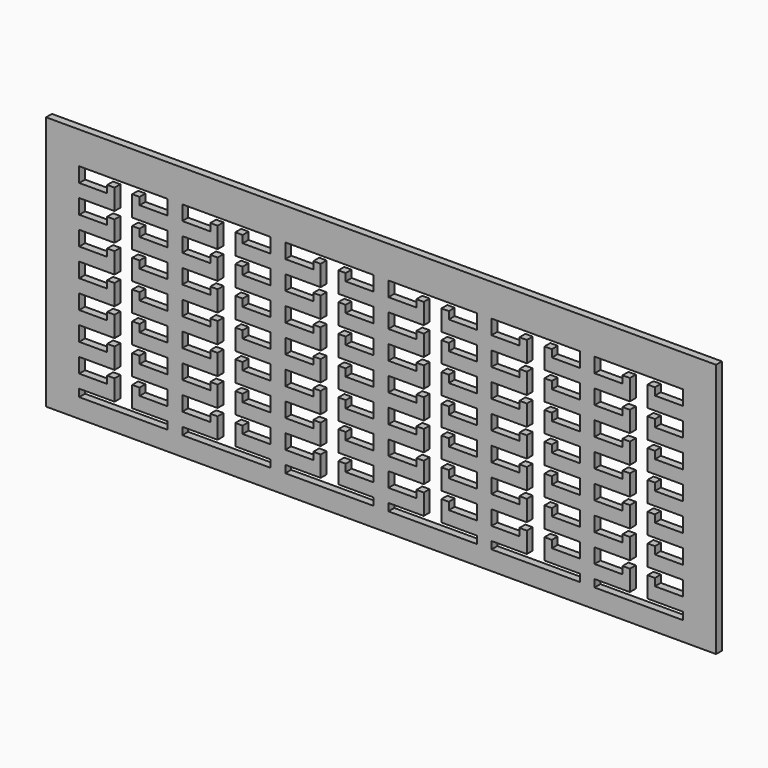
from build123d import *

# Parameters (mm, degrees)
F0_W     = 577.85
F0_H     = 219.71
F1_DEPTH = 6.35


# Not quite as in the source:
# - ends of sketch curves that miss each other by under 0.0002 mm in the source are joined


with BuildPart() as f1:
    # F0 (on Front) → F1 (new body)
    with BuildSketch(Plane.XZ):
        with Locations((-282.1097705345, 13.2987275338)):
            Rectangle(F0_W, F0_H)
        Polygon((-542.4597705345, -62.2027724662), (-542.4597705345, -49.5027724662), (-511.9797705345, -49.5027724662), (-511.9797705345, -31.7227724662), (-518.3297705345, -31.7227724662), (-518.3297705345, -38.0727724662), (-542.4597705345, -38.0727724662), (-542.4597705345, -25.3727724662), (-511.9797705345, -25.3727724662), (-511.9797705345, -7.5927724662), (-518.3297705345, -7.5927724662), (-518.3297705345, -13.9427724662), (-542.4597705345, -13.9427724662), (-542.4597705345, -1.2427724662), (-511.9797705345, -1.2427724662), (-511.9797705345, 16.5372275338), (-518.3297705345, 16.5372275338), (-518.3297705345, 10.1872275338), (-542.4597705345, 10.1872275338), (-542.4597705345, 22.8872275338), (-511.9797705345, 22.8872275338), (-511.9797705345, 40.6672275338), (-518.3297705345, 40.6672275338), (-518.3297705345, 34.3172275338), (-542.4597705345, 34.3172275338), (-542.4597705345, 47.0172275338), (-511.9797705345, 47.0172275338), (-511.9797705345, 64.7972275338), (-518.3297705345, 64.7972275338), (-518.3297705345, 58.4472275338), (-542.4597705345, 58.4472275338), (-542.4597705345, 71.1472275338), (-511.9797705345, 71.1472275338), (-511.9797705345, 88.9272173567), (-518.3297705345, 88.9272173567), (-518.3297705345, 82.5772173567), (-542.4597705345, 82.5772173567), (-542.4597705345, 95.2772173567), (-466.2597705346, 95.2772173567), (-466.2597705346, 82.5772173567), (-490.3897705345, 82.5772173567), (-490.3897705345, 88.9272173567), (-496.7397705346, 88.9272173567), (-496.7397705346, 71.1472173567), (-466.2597705346, 71.1472173568), (-466.2597705346, 58.4472173568), (-490.3897705346, 58.4472173568), (-490.3897705346, 64.7972173568), (-496.7397705346, 64.7972173568), (-496.7397705346, 47.0172173567), (-466.2597705346, 47.0172173567), (-466.2597705345, 34.3172275338), (-490.3897705345, 34.3172275338), (-490.3897705345, 40.6672275338), (-496.7397705345, 40.6672275338), (-496.7397705345, 22.8872275338), (-466.2597705345, 22.8872275338), (-466.2597705345, 10.1872275338), (-490.3897705345, 10.1872275338), (-490.3897705345, 16.5372275338), (-496.7397705345, 16.5372275338), (-496.7397705345, -1.2427724662), (-466.2597705345, -1.2427724662), (-466.2597705345, -13.9427724662), (-490.3897705345, -13.9427724662), (-490.3897705345, -7.5927724662), (-496.7397705345, -7.5927724662), (-496.7397705345, -25.3727724662), (-466.2597705345, -25.3727724662), (-466.2597705345, -38.0727724662), (-490.3897705345, -38.0727724662), (-490.3897705345, -31.7227724662), (-496.7397705345, -31.7227724662), (-496.7397705345, -49.5027724662), (-466.2597705345, -49.5027724662), (-466.2597705345, -62.2027724662), (-490.3897705345, -62.2027724662), (-490.3897705345, -55.8527724662), (-496.7397705345, -55.8527724662), (-496.7397705345, -73.6327724662), (-466.2597705345, -73.6327724662), (-466.2597705345, -80.0462724662), (-542.4597705345, -80.0462724662), (-542.4597705345, -73.6327724662), (-511.9797705345, -73.6327724662), (-511.9797705345, -55.8527724662), (-518.3297705345, -55.8527724662), (-518.3297705345, -62.2027724662), align=None, mode=Mode.SUBTRACT)
        Polygon((-453.5597705345, -62.2027724662), (-453.5597705345, -49.5027724662), (-423.0797705345, -49.5027724662), (-423.0797705345, -31.7227724662), (-429.4297705345, -31.7227724662), (-429.4297705345, -38.0727724662), (-453.5597705345, -38.0727724662), (-453.5597705345, -25.3727724662), (-423.0797705345, -25.3727724662), (-423.0797705345, -7.5927724662), (-429.4297705345, -7.5927724662), (-429.4297705345, -13.9427724662), (-453.5597705345, -13.9427724662), (-453.5597705345, -1.2427724662), (-423.0797705345, -1.2427724662), (-423.0797705345, 16.5372275338), (-429.4297705345, 16.5372275338), (-429.4297705345, 10.1872275338), (-453.5597705345, 10.1872275338), (-453.5597705345, 22.8872275338), (-423.0797705345, 22.8872275338), (-423.0797705345, 40.6672275338), (-429.4297705345, 40.6672275338), (-429.4297705345, 34.3172275338), (-453.5597705345, 34.3172275338), (-453.5597705345, 47.0172275338), (-423.0797705345, 47.0172275338), (-423.0797705345, 64.7972275338), (-429.4297705345, 64.7972275338), (-429.4297705345, 58.4472275338), (-453.5597705345, 58.4472275338), (-453.5597705345, 71.1472275338), (-423.0797705345, 71.1472275338), (-423.0797705345, 88.9272275338), (-429.4297705345, 88.9272275338), (-429.4297705345, 82.5772275338), (-453.5597705345, 82.5772275338), (-453.5597705345, 95.2772275338), (-377.3597705345, 95.2772275338), (-377.3597705345, 82.5772275338), (-401.4897705345, 82.5772275338), (-401.4897705345, 88.9272275338), (-407.8397705345, 88.9272275338), (-407.8397705345, 71.1472275338), (-377.3597705345, 71.1472275338), (-377.3597705345, 58.4472275338), (-401.4897705345, 58.4472275338), (-401.4897705345, 64.7972275338), (-407.8397705345, 64.7972275338), (-407.8397705345, 47.0172275338), (-377.3597705345, 47.0172275338), (-377.3597705345, 34.3172275338), (-401.4897705345, 34.3172275338), (-401.4897705345, 40.6672275338), (-407.8397705345, 40.6672275338), (-407.8397705345, 22.8872275338), (-377.3597705345, 22.8872275338), (-377.3597705345, 10.1872275338), (-401.4897705345, 10.1872275338), (-401.4897705345, 16.5372275338), (-407.8397705345, 16.5372275338), (-407.8397705345, -1.2427724662), (-377.3597705345, -1.2427724662), (-377.3597705345, -13.9427724662), (-401.4897705345, -13.9427724662), (-401.4897705345, -7.5927724662), (-407.8397705345, -7.5927724662), (-407.8397705345, -25.3727724662), (-377.3597705345, -25.3727724662), (-377.3597705345, -38.0727724662), (-401.4897705345, -38.0727724662), (-401.4897705345, -31.7227724662), (-407.8397705345, -31.7227724662), (-407.8397705345, -49.5027724662), (-377.3597705345, -49.5027724662), (-377.3597705345, -62.2027724662), (-401.4897705345, -62.2027724662), (-401.4897705345, -55.8527724662), (-407.8397705345, -55.8527724662), (-407.8397705345, -73.6327724662), (-377.3597705345, -73.6327724662), (-377.3597705345, -80.0462724662), (-453.5597705345, -80.0462724662), (-453.5597705345, -73.6327724662), (-423.0797705345, -73.6327724662), (-423.0797705345, -55.8527724662), (-429.4297705345, -55.8527724662), (-429.4297705345, -62.2027724662), align=None, mode=Mode.SUBTRACT)
        Polygon((-364.6597705345, -62.2027724662), (-364.6597705345, -49.5027724662), (-334.1797705345, -49.5027724662), (-334.1797705345, -31.7227724662), (-340.5297705345, -31.7227724662), (-340.5297705345, -38.0727724662), (-364.6597705345, -38.0727724662), (-364.6597705345, -25.3727724662), (-334.1797705345, -25.3727724662), (-334.1797705345, -7.5927724662), (-340.5297705345, -7.5927724662), (-340.5297705345, -13.9427724662), (-364.6597705345, -13.9427724662), (-364.6597705345, -1.2427724662), (-334.1797705345, -1.2427724662), (-334.1797705345, 16.5372275338), (-340.5297705345, 16.5372275338), (-340.5297705345, 10.1872275338), (-364.6597705345, 10.1872275338), (-364.6597705345, 22.8872275338), (-334.1797705345, 22.8872275338), (-334.1797705345, 40.6672275338), (-340.5297705345, 40.6672275338), (-340.5297705345, 34.3172275338), (-364.6597705345, 34.3172275338), (-364.6597705345, 47.0172275338), (-334.1797705345, 47.0172275338), (-334.1797705345, 64.7972275338), (-340.5297705345, 64.7972275338), (-340.5297705345, 58.4472275338), (-364.6597705345, 58.4472275338), (-364.6597705345, 71.1472275338), (-334.1797705345, 71.1472275338), (-334.1797705345, 88.9272275338), (-340.5297705345, 88.9272275338), (-340.5297705345, 82.5772275338), (-364.6597705345, 82.5772275338), (-364.6597705345, 95.2772275338), (-288.4597705345, 95.2772275338), (-288.4597705345, 82.5772275338), (-312.5897705345, 82.5772275338), (-312.5897705345, 88.9272275338), (-318.9397705345, 88.9272275338), (-318.9397705345, 71.1472275338), (-288.4597705346, 71.1472275338), (-288.4597705346, 58.4472275338), (-312.5897705346, 58.4472275338), (-312.5897705346, 64.7972275338), (-318.9397705345, 64.7972275338), (-318.9397705346, 47.0172275338), (-288.4597705346, 47.0172275338), (-288.4597705345, 34.3172275338), (-312.5897705345, 34.3172275338), (-312.5897705345, 40.6672275338), (-318.9397705345, 40.6672275338), (-318.9397705345, 22.8872275338), (-288.4597705345, 22.8872275338), (-288.4597705345, 10.1872275338), (-312.5897705345, 10.1872275338), (-312.5897705345, 16.5372275338), (-318.9397705345, 16.5372275338), (-318.9397705345, -1.2427724662), (-288.4597705345, -1.2427724662), (-288.4597705345, -13.9427724662), (-312.5897705345, -13.9427724662), (-312.5897705345, -7.5927724662), (-318.9397705345, -7.5927724662), (-318.9397705345, -25.3727724662), (-288.4597705345, -25.3727724662), (-288.4597705345, -38.0727724662), (-312.5897705345, -38.0727724662), (-312.5897705345, -31.7227724662), (-318.9397705345, -31.7227724662), (-318.9397705345, -49.5027724662), (-288.4597705345, -49.5027724662), (-288.4597705345, -62.2027724662), (-312.5897705345, -62.2027724662), (-312.5897705345, -55.8527724662), (-318.9397705345, -55.8527724662), (-318.9397705345, -73.6327724662), (-288.4597705345, -73.6327724662), (-288.4597705345, -80.0462724662), (-364.6597705345, -80.0462724662), (-364.6597705345, -73.6327724662), (-334.1797705345, -73.6327724662), (-334.1797705345, -55.8527724662), (-340.5297705345, -55.8527724662), (-340.5297705345, -62.2027724662), align=None, mode=Mode.SUBTRACT)
        Polygon((-275.7597705345, -62.2027724662), (-275.7597705345, -49.5027724662), (-245.2797705345, -49.5027724662), (-245.2797705345, -31.7227724662), (-251.6297705345, -31.7227724662), (-251.6297705345, -38.0727724662), (-275.7597705345, -38.0727724662), (-275.7597705345, -25.3727724662), (-245.2797705345, -25.3727724662), (-245.2797705345, -7.5927724662), (-251.6297705345, -7.5927724662), (-251.6297705345, -13.9427724662), (-275.7597705345, -13.9427724662), (-275.7597705345, -1.2427724662), (-245.2797705345, -1.2427724662), (-245.2797705345, 16.5372275338), (-251.6297705345, 16.5372275338), (-251.6297705345, 10.1872275338), (-275.7597705345, 10.1872275338), (-275.7597705345, 22.8872275338), (-245.2797705345, 22.8872275338), (-245.2797705345, 40.6672275338), (-251.6297705345, 40.6672275338), (-251.6297705345, 34.3172275338), (-275.7597705345, 34.3172275338), (-275.7597705345, 47.0172275338), (-245.2797705345, 47.0172275338), (-245.2797705345, 64.7972275338), (-251.6297705345, 64.7972275338), (-251.6297705345, 58.4472275338), (-275.7597705345, 58.4472275338), (-275.7597705345, 71.1472275338), (-245.2797705345, 71.1472275338), (-245.2797705345, 88.9272275338), (-251.6297705345, 88.9272275338), (-251.6297705345, 82.5772275338), (-275.7597705345, 82.5772275338), (-275.7597705345, 95.2772275338), (-199.5597705345, 95.2772275338), (-199.5597705345, 82.5772275338), (-223.6897705345, 82.5772275338), (-223.6897705345, 88.9272275338), (-230.0397705345, 88.9272275338), (-230.0397705345, 71.1472275338), (-199.5597705345, 71.1472275338), (-199.5597705345, 58.4472275338), (-223.6897705345, 58.4472275338), (-223.6897705345, 64.7972275338), (-230.0397705345, 64.7972275338), (-230.0397705345, 47.0172275338), (-199.5597705345, 47.0172275338), (-199.5597705345, 34.3172275338), (-223.6897705345, 34.3172275338), (-223.6897705345, 40.6672275338), (-230.0397705345, 40.6672275338), (-230.0397705345, 22.8872275338), (-199.5597705345, 22.8872275338), (-199.5597705345, 10.1872275338), (-223.6897705345, 10.1872275338), (-223.6897705345, 16.5372275338), (-230.0397705345, 16.5372275338), (-230.0397705345, -1.2427724662), (-199.5597705345, -1.2427724662), (-199.5597705345, -13.9427724662), (-223.6897705345, -13.9427724662), (-223.6897705345, -7.5927724662), (-230.0397705345, -7.5927724662), (-230.0397705345, -25.3727724662), (-199.5597705345, -25.3727724662), (-199.5597705345, -38.0727724662), (-223.6897705345, -38.0727724662), (-223.6897705345, -31.7227724662), (-230.0397705345, -31.7227724662), (-230.0397705345, -49.5027724662), (-199.5597705345, -49.5027724662), (-199.5597705345, -62.2027724662), (-223.6897705345, -62.2027724662), (-223.6897705345, -55.8527724662), (-230.0397705345, -55.8527724662), (-230.0397705345, -73.6327724662), (-199.5597705345, -73.6327724662), (-199.5597705345, -80.0462724662), (-275.7597705345, -80.0462724662), (-275.7597705345, -73.6327724662), (-245.2797705345, -73.6327724662), (-245.2797705345, -55.8527724662), (-251.6297705345, -55.8527724662), (-251.6297705345, -62.2027724662), align=None, mode=Mode.SUBTRACT)
        Polygon((-186.8597705345, -62.2027724662), (-186.8597705345, -49.5027724662), (-156.3797705345, -49.5027724662), (-156.3797705345, -31.7227724662), (-162.7297705345, -31.7227724662), (-162.7297705345, -38.0727724662), (-186.8597705345, -38.0727724662), (-186.8597705345, -25.3727724662), (-156.3797705345, -25.3727724662), (-156.3797705345, -7.5927724662), (-162.7297705345, -7.5927724662), (-162.7297705345, -13.9427724662), (-186.8597705345, -13.9427724662), (-186.8597705345, -1.2427724662), (-156.3797705345, -1.2427724662), (-156.3797705345, 16.5372275338), (-162.7297705345, 16.5372275338), (-162.7297705345, 10.1872275338), (-186.8597705345, 10.1872275338), (-186.8597705345, 22.8872275338), (-156.3797705345, 22.8872275338), (-156.3797705345, 40.6672275338), (-162.7297705345, 40.6672275338), (-162.7297705345, 34.3172275338), (-186.8597705345, 34.3172275338), (-186.8597705345, 47.0172275338), (-156.3797705345, 47.0172275338), (-156.3797705345, 64.7972275338), (-162.7297705345, 64.7972275338), (-162.7297705345, 58.4472275338), (-186.8597705345, 58.4472275338), (-186.8597705345, 71.1472275338), (-156.3797705345, 71.1472275338), (-156.3797705345, 88.9272275338), (-162.7297705345, 88.9272275338), (-162.7297705345, 82.5772275338), (-186.8597705345, 82.5772275338), (-186.8597705345, 95.2772275338), (-110.6597705345, 95.2772275338), (-110.6597705345, 82.5772275338), (-134.7897705345, 82.5772275338), (-134.7897705345, 88.9272275338), (-141.1397705345, 88.9272275338), (-141.1397705345, 71.1472275338), (-110.6597705345, 71.1472275338), (-110.6597705345, 58.4472275338), (-134.7897705345, 58.4472275338), (-134.7897705345, 64.7972275338), (-141.1397705345, 64.7972275338), (-141.1397705345, 47.0172275338), (-110.6597705345, 47.0172275338), (-110.6597705345, 34.3172275338), (-134.7897705345, 34.3172275338), (-134.7897705345, 40.6672275338), (-141.1397705345, 40.6672275338), (-141.1397705345, 22.8872275338), (-110.6597705345, 22.8872275338), (-110.6597705345, 10.1872275338), (-134.7897705345, 10.1872275338), (-134.7897705345, 16.5372275338), (-141.1397705345, 16.5372275338), (-141.1397705345, -1.2427724662), (-110.6597705345, -1.2427724662), (-110.6597705345, -13.9427724662), (-134.7897705345, -13.9427724662), (-134.7897705345, -7.5927724662), (-141.1397705345, -7.5927724662), (-141.1397705345, -25.3727724662), (-110.6597705345, -25.3727724662), (-110.6597705345, -38.0727724662), (-134.7897705345, -38.0727724662), (-134.7897705345, -31.7227724662), (-141.1397705345, -31.7227724662), (-141.1397705345, -49.5027724662), (-110.6597705345, -49.5027724662), (-110.6597705345, -62.2027724662), (-134.7897705345, -62.2027724662), (-134.7897705345, -55.8527724662), (-141.1397705345, -55.8527724662), (-141.1397705345, -73.6327724662), (-110.6597705345, -73.6327724662), (-110.6597705345, -80.0462724662), (-186.8597705345, -80.0462724662), (-186.8597705345, -73.6327724662), (-156.3797705345, -73.6327724662), (-156.3797705345, -55.8527724662), (-162.7297705345, -55.8527724662), (-162.7297705345, -62.2027724662), align=None, mode=Mode.SUBTRACT)
        Polygon((-97.9597705345, -62.2027724662), (-97.9597705345, -49.5027724662), (-67.4797705345, -49.5027724662), (-67.4797705345, -31.7227724662), (-73.8297705345, -31.7227724662), (-73.8297705345, -38.0727724662), (-97.9597705345, -38.0727724662), (-97.9597705345, -25.3727724662), (-67.4797705345, -25.3727724662), (-67.4797705345, -7.5927724662), (-73.8297705345, -7.5927724662), (-73.8297705345, -13.9427724662), (-97.9597705345, -13.9427724662), (-97.9597705345, -1.2427724662), (-67.4797705345, -1.2427724662), (-67.4797705345, 16.5372275338), (-73.8297705345, 16.5372275338), (-73.8297705345, 10.1872275338), (-97.9597705345, 10.1872275338), (-97.9597705345, 22.8872275338), (-67.4797705345, 22.8872275338), (-67.4797705345, 40.6672275338), (-73.8297705345, 40.6672275338), (-73.8297705345, 34.3172275338), (-97.9597705345, 34.3172275338), (-97.9597705345, 47.0172275338), (-67.4797705345, 47.0172275338), (-67.4797705345, 64.7972275338), (-73.8297705345, 64.7972275338), (-73.8297705345, 58.4472275338), (-97.9597705345, 58.4472275338), (-97.9597705345, 71.1472275338), (-67.4797705345, 71.1472275338), (-67.4797705345, 88.9272275338), (-73.8297705345, 88.9272275338), (-73.8297705345, 82.5772275338), (-97.9597705345, 82.5772275338), (-97.9597705345, 95.2772275338), (-21.7597705345, 95.2772275338), (-21.7597705345, 82.5772275338), (-45.8897705345, 82.5772275338), (-45.8897705345, 88.9272275338), (-52.2397705345, 88.9272275338), (-52.2397705345, 71.1472275338), (-21.7597705345, 71.1472275338), (-21.7597705345, 58.4472275338), (-45.8897705345, 58.4472275338), (-45.8897705345, 64.7972275338), (-52.2397705345, 64.7972275338), (-52.2397705345, 47.0172275338), (-21.7597705345, 47.0172275338), (-21.7597705345, 34.3172275338), (-45.8897705345, 34.3172275338), (-45.8897705345, 40.6672275338), (-52.2397705345, 40.6672275338), (-52.2397705345, 22.8872275338), (-21.7597705345, 22.8872275338), (-21.7597705345, 10.1872275338), (-45.8897705345, 10.1872275338), (-45.8897705345, 16.5372275338), (-52.2397705345, 16.5372275338), (-52.2397705345, -1.2427724662), (-21.7597705345, -1.2427724662), (-21.7597705345, -13.9427724662), (-45.8897705345, -13.9427724662), (-45.8897705345, -7.5927724662), (-52.2397705345, -7.5927724662), (-52.2397705345, -25.3727724662), (-21.7597705345, -25.3727724662), (-21.7597705345, -38.0727724662), (-45.8897705345, -38.0727724662), (-45.8897705345, -31.7227724662), (-52.2397705345, -31.7227724662), (-52.2397705345, -49.5027724662), (-21.7597705345, -49.5027724662), (-21.7597705345, -62.2027724662), (-45.8897705345, -62.2027724662), (-45.8897705345, -55.8527724662), (-52.2397705345, -55.8527724662), (-52.2397705345, -73.6327724662), (-21.7597705345, -73.6327724662), (-21.7597705345, -80.0462724662), (-97.9597705345, -80.0462724662), (-97.9597705345, -73.6327724662), (-67.4797705345, -73.6327724662), (-67.4797705345, -55.8527724662), (-73.8297705345, -55.8527724662), (-73.8297705345, -62.2027724662), align=None, mode=Mode.SUBTRACT)
    extrude(amount=F1_DEPTH)


solid = f1.part
